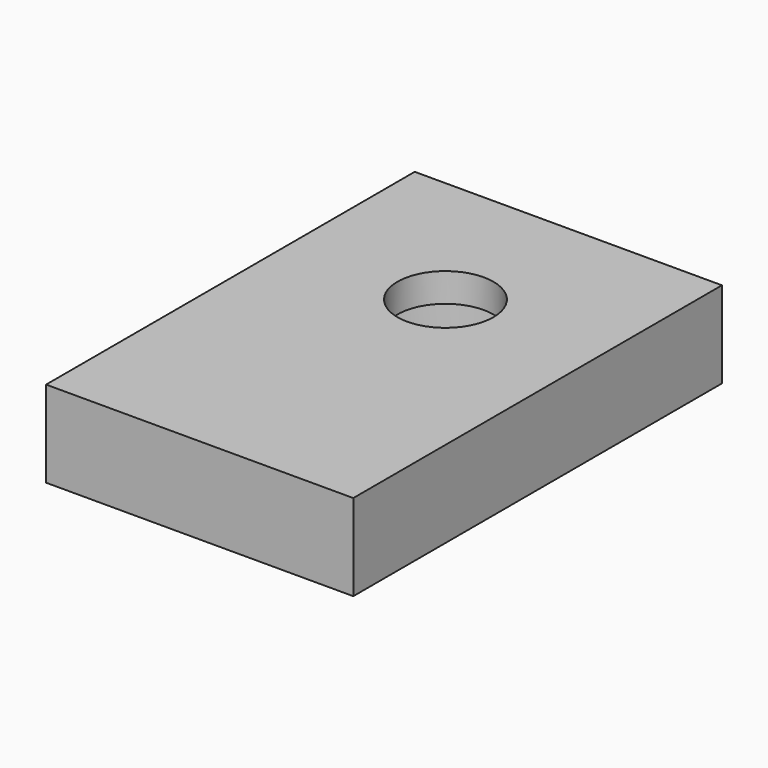
from build123d import *

# Parameters (mm, degrees)
F0_W     = 25.4
F0_H     = 38.1
F1_DEPTH = 4.7625
F2_W     = 25.4
F2_H     = 38.1
F2_R     = 3.96875
F3_DEPTH = 2.38125


# Not quite as in the source:
# - a length typed as a fraction of an inch, garbled in the dataset ("3 / 203.2 mm" for 3/8 in), is restored


with BuildPart() as f1:
    # F0 (on Top) → F1 (new body)
    with BuildSketch(Plane.XY):
        with Locations((0, -6.35)):
            Rectangle(F0_W, F0_H)
        with BuildLine():
            ThreePointArc((-8.73125, 0), (0, 8.73125), (8.73125, 0))
            Line((8.73125, 0), (8.73125, -19.05))
            Line((8.73125, -19.05), (-8.73125, -19.05))
            Line((-8.73125, -19.05), (-8.73125, 0))
        make_face(mode=Mode.SUBTRACT)
    extrude(amount=F1_DEPTH)

    # F2 (on face) → F3 (join)
    with BuildSketch(Plane.XY.offset(4.7625)):
        with Locations((0, -6.35)):
            Rectangle(F2_W, F2_H)
        Circle(F2_R, mode=Mode.SUBTRACT)
    extrude(amount=F3_DEPTH)


solid = f1.part
